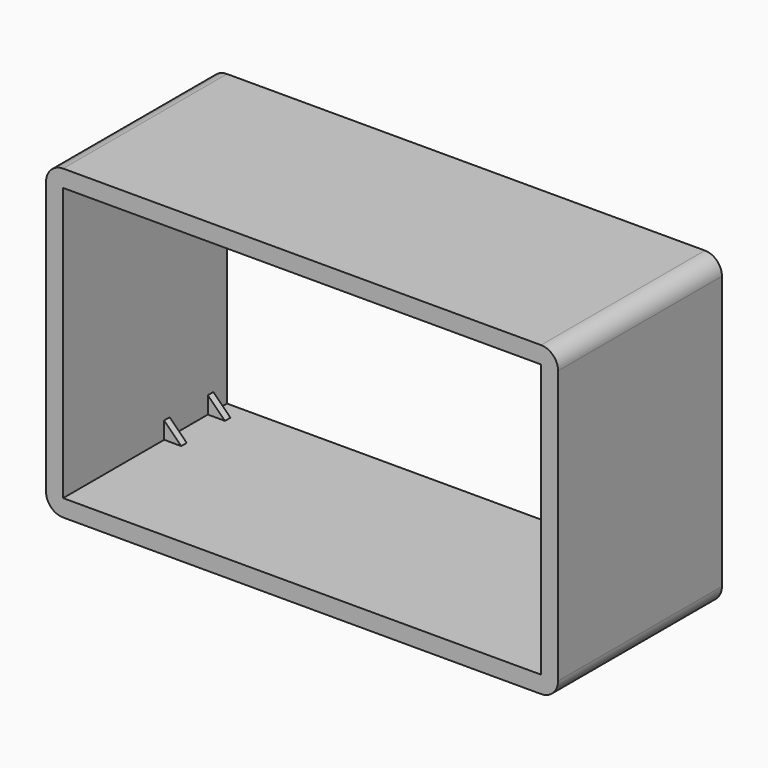
from build123d import *

# Parameters (mm, degrees)
F0_W     = 1500
F0_H     = 900
F0_W_2   = 1400
F0_H_2   = 800
F1_DEPTH = 600
F2_SCALE = 0.1
F6_DEPTH = 2
F7_R     = 5


# Not quite as in the source:
# - a pattern or mirror of a feature is missing from the dataset's text; its kind, count and spacing are read off the source's solid


with BuildPart() as f1:
    # F0 (on Front) → F1 (new body)
    with BuildSketch(Plane.XZ):
        Rectangle(F0_W, F0_H)
        Rectangle(F0_W_2, F0_H_2, mode=Mode.SUBTRACT)
    extrude(amount=F1_DEPTH)


with BuildPart() as f1_1:
    # F2: moved
    add(f1.part.scale(F2_SCALE))

    # F5 (on offset) → F6 (join)
    with BuildSketch(Plane(origin=(0, -21, 0), x_dir=(-1, 0, 0), z_dir=(0, 1, 0))):
        Polygon((-65, 40), (-70, 40), (-70, 35), align=None)
        Polygon((65, 40), (70, 35), (70, 40), align=None)
        Polygon((-70, -35), (-70, -40), (-65, -40), align=None)
        Polygon((65, -40), (70, -40), (70, -35), align=None)
    f6 = extrude(amount=-F6_DEPTH)

    # F6_copies: F6 across plane
    add(f6.mirror(Plane.ZX.offset(-14)))

    # F7
    f7_edges = [f1_1.edges().sort_by_distance(p)[0] for p in [
        (75, -30, 45),
        (75, -30, -45),
        (-75, -30, -45),
        (-75, -30, 45),
    ]]
    fillet(f7_edges, radius=F7_R)


solid = f1_1.part
